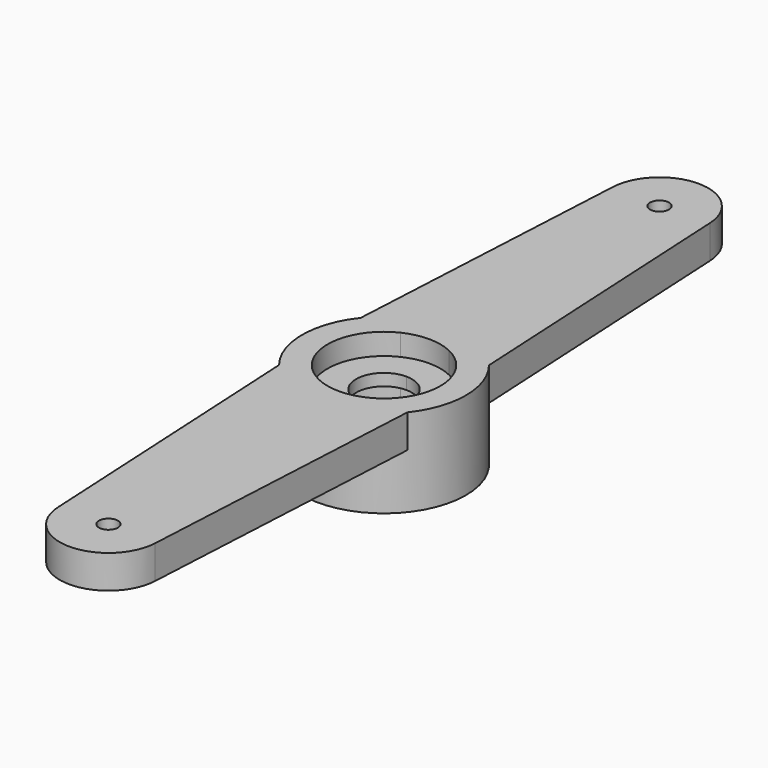
from build123d import *

# Parameters (mm, degrees)
F0_R     = 0.4
F1_DEPTH = 1.4
F2_DEPTH = 2.3
F3_DEPTH = 0.5


with BuildPart() as f1:
    # F0 (on Top) → F1 (new body)
    with BuildSketch(Plane.XY):
        with BuildLine():
            ThreePointArc((2.7, -2.1476731595), (3.2571076126, -1.1374313166), (3.45, 0))
            ThreePointArc((3.45, 0), (3.2571076126, 1.1374313166), (2.7, 2.1476731595))
            Line((2.7, 2.1476731595), (1.0139649895, 2.1476731595))
            ThreePointArc((1.0139649895, 2.1476731595), (2.0060897101, 1.2713099838), (2.375, 0))
            ThreePointArc((2.375, 0), (2.0060897101, -1.2713099838), (1.0139649895, -2.1476731595))
            Line((1.0139649895, -2.1476731595), (2.7, -2.1476731595))
        make_face()
        with BuildLine():
            Line((1.0139649895, 2.1476731595), (2.7, 2.1476731595))
            ThreePointArc((2.7, 2.1476731595), (0, 3.45), (-2.7, 2.1476731595))
            Line((-2.7, 2.1476731595), (-1.0139649895, 2.1476731595))
            ThreePointArc((-1.0139649895, 2.1476731595), (0, 2.375), (1.0139649895, 2.1476731595))
        make_face()
        with BuildLine():
            ThreePointArc((-2.7, 2.1476731595), (0, 3.45), (2.7, 2.1476731595))
            Line((2.7, 2.1476731595), (2.0471920173, 14.6072606371))
            ThreePointArc((2.0471920173, 14.6072606371), (2.0492978841, 14.553648693), (2.05, 14.5))
            ThreePointArc((2.05, 14.5), (-0.053648693, 12.4507021159), (-2.0471920173, 14.6072606371))
            Line((-2.0471920173, 14.6072606371), (-2.7, 2.1476731595))
        make_face()
        with BuildLine():
            Line((2.0471920173, -14.6072606371), (2.7, -2.1476731595))
            ThreePointArc((2.7, -2.1476731595), (0, -3.45), (-2.7, -2.1476731595))
            Line((-2.7, -2.1476731595), (-2.0471920173, -14.6072606371))
            ThreePointArc((-2.0471920173, -14.6072606371), (-0.053648693, -12.4507021159), (2.05, -14.5))
            ThreePointArc((2.05, -14.5), (2.0492978841, -14.553648693), (2.0471920173, -14.6072606371))
        make_face()
        with BuildLine():
            ThreePointArc((-2.7, -2.1476731595), (0, -3.45), (2.7, -2.1476731595))
            Line((2.7, -2.1476731595), (1.0139649895, -2.1476731595))
            ThreePointArc((1.0139649895, -2.1476731595), (0, -2.375), (-1.0139649895, -2.1476731595))
            Line((-1.0139649895, -2.1476731595), (-2.7, -2.1476731595))
        make_face()
        with BuildLine():
            Line((-1.0139649895, 2.1476731595), (-2.7, 2.1476731595))
            ThreePointArc((-2.7, 2.1476731595), (-3.45, 0), (-2.7, -2.1476731595))
            Line((-2.7, -2.1476731595), (-1.0139649895, -2.1476731595))
            ThreePointArc((-1.0139649895, -2.1476731595), (-2.375, 0), (-1.0139649895, 2.1476731595))
        make_face()
        with BuildLine():
            ThreePointArc((2.05, 14.5), (2.0492978841, 14.553648693), (2.0471920173, 14.6072606371))
            ThreePointArc((2.0471920173, 14.6072606371), (0, 16.55), (-2.0471920173, 14.6072606371))
            ThreePointArc((-2.0471920173, 14.6072606371), (-0.053648693, 12.4507021159), (2.05, 14.5))
        make_face()
        with Locations((0, 14.5)):
            Circle(F0_R, mode=Mode.SUBTRACT)
        with BuildLine():
            ThreePointArc((-2.0471920173, -14.6072606371), (0, -16.55), (2.0471920173, -14.6072606371))
            ThreePointArc((2.0471920173, -14.6072606371), (2.0492978841, -14.553648693), (2.05, -14.5))
            ThreePointArc((2.05, -14.5), (-0.053648693, -12.4507021159), (-2.0471920173, -14.6072606371))
        make_face()
        with Locations((0, -14.5)):
            Circle(F0_R, mode=Mode.SUBTRACT)
    extrude(amount=F1_DEPTH)

    # F0 (on Top) → F2 (join)
    with BuildSketch(Plane.XY):
        with BuildLine():
            Line((-1.0139649895, 2.1476731595), (-2.7, 2.1476731595))
            ThreePointArc((-2.7, 2.1476731595), (-3.45, 0), (-2.7, -2.1476731595))
            Line((-2.7, -2.1476731595), (-1.0139649895, -2.1476731595))
            ThreePointArc((-1.0139649895, -2.1476731595), (-2.375, 0), (-1.0139649895, 2.1476731595))
        make_face()
        with BuildLine():
            Line((1.0139649895, 2.1476731595), (2.7, 2.1476731595))
            ThreePointArc((2.7, 2.1476731595), (0, 3.45), (-2.7, 2.1476731595))
            Line((-2.7, 2.1476731595), (-1.0139649895, 2.1476731595))
            ThreePointArc((-1.0139649895, 2.1476731595), (0, 2.375), (1.0139649895, 2.1476731595))
        make_face()
        with BuildLine():
            ThreePointArc((-2.7, -2.1476731595), (0, -3.45), (2.7, -2.1476731595))
            Line((2.7, -2.1476731595), (1.0139649895, -2.1476731595))
            ThreePointArc((1.0139649895, -2.1476731595), (0, -2.375), (-1.0139649895, -2.1476731595))
            Line((-1.0139649895, -2.1476731595), (-2.7, -2.1476731595))
        make_face()
        with BuildLine():
            ThreePointArc((2.7, -2.1476731595), (3.2571076126, -1.1374313166), (3.45, 0))
            ThreePointArc((3.45, 0), (3.2571076126, 1.1374313166), (2.7, 2.1476731595))
            Line((2.7, 2.1476731595), (1.0139649895, 2.1476731595))
            ThreePointArc((1.0139649895, 2.1476731595), (2.0060897101, 1.2713099838), (2.375, 0))
            ThreePointArc((2.375, 0), (2.0060897101, -1.2713099838), (1.0139649895, -2.1476731595))
            Line((1.0139649895, -2.1476731595), (2.7, -2.1476731595))
        make_face()
    extrude(amount=-F2_DEPTH)

    # F0 (on Top) → F3 (join)
    with BuildSketch(Plane.XY):
        with BuildLine():
            Line((0, 2.1476731595), (1.0139649895, 2.1476731595))
            ThreePointArc((1.0139649895, 2.1476731595), (0, 2.375), (-1.0139649895, 2.1476731595))
            Line((-1.0139649895, 2.1476731595), (0, 2.1476731595))
        make_face()
        with BuildLine():
            ThreePointArc((2.375, 0), (2.0060897101, 1.2713099838), (1.0139649895, 2.1476731595))
            Line((1.0139649895, 2.1476731595), (0, 2.1476731595))
            Line((0, 2.1476731595), (-1.0139649895, 2.1476731595))
            ThreePointArc((-1.0139649895, 2.1476731595), (-2.375, 0), (-1.0139649895, -2.1476731595))
            Line((-1.0139649895, -2.1476731595), (1.0139649895, -2.1476731595))
            ThreePointArc((1.0139649895, -2.1476731595), (2.0060897101, -1.2713099838), (2.375, 0))
        make_face()
        with BuildLine():
            ThreePointArc((1.175, 0), (-0.8308504679, -0.8308504679), (0, 1.175))
            ThreePointArc((0, 1.175), (0.8308504679, 0.8308504679), (1.175, 0))
        make_face(mode=Mode.SUBTRACT)
        with BuildLine():
            ThreePointArc((-1.0139649895, -2.1476731595), (0, -2.375), (1.0139649895, -2.1476731595))
            Line((1.0139649895, -2.1476731595), (-1.0139649895, -2.1476731595))
        make_face()
    extrude(amount=F3_DEPTH)


solid = f1.part
